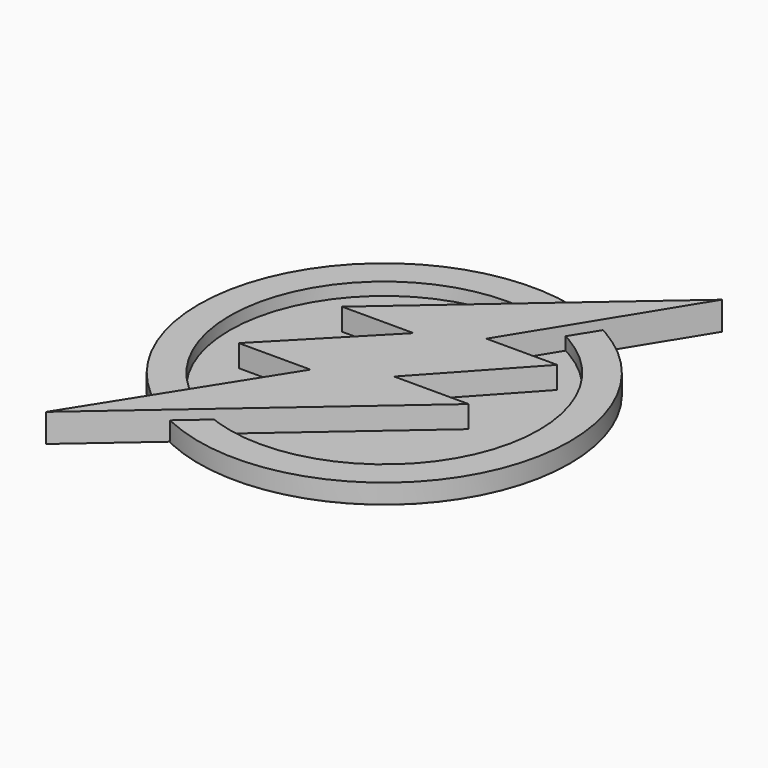
from build123d import *

# Parameters (mm, degrees)
F1_R     = 30
F1_R_2   = 25
F5_DEPTH = 1
F6_DEPTH = 0.1
F7_DEPTH = 3.048
F8_DEPTH = 4.572


# Not quite as in the source:
# - the program builds the solid bodies; features that only make, move or delete a surface that nothing else refers to are left out


with BuildPart() as f5:
    # F1 (on face) → F5 (new body)
    with BuildSketch(Plane.XY):
        Circle(F1_R)
        Circle(F1_R_2, mode=Mode.SUBTRACT)
        Circle(F1_R_2)
    extrude(amount=F5_DEPTH)


with BuildPart() as f6:
    # F1 (on face) → F6 (new body)
    with BuildSketch(Plane.XY):
        Circle(F1_R)
        Circle(F1_R_2, mode=Mode.SUBTRACT)
        Circle(F1_R_2)
    extrude(amount=-F6_DEPTH)


with BuildPart() as f7:
    # F1 (on face) → F7 (new body)
    with BuildSketch(Plane.XY):
        Circle(F1_R)
        Circle(F1_R_2, mode=Mode.SUBTRACT)
    extrude(amount=F7_DEPTH)


with BuildPart() as f8:
    # F2 (on Top) → F8 (new body)
    with BuildSketch(Plane.XY):
        Polygon((6.0379398285, 13.0822043866), (22.5992734988, 39.9943725895), (-13.6509970043, 8.5318721831), (-2.0855690818, 8.5318721831), (-17.6184918681, -7.3942895979), (-6.025892119, -7.3942895979), (-24.8665944569, -37.2795380606), (15.4645281288, -2.2751658689), (3.412750084, -2.2751658689), (17.4903385899, 13.0822043866), align=None)
    extrude(amount=F8_DEPTH)


solid = Compound([f5.part, f6.part, f7.part, f8.part])
